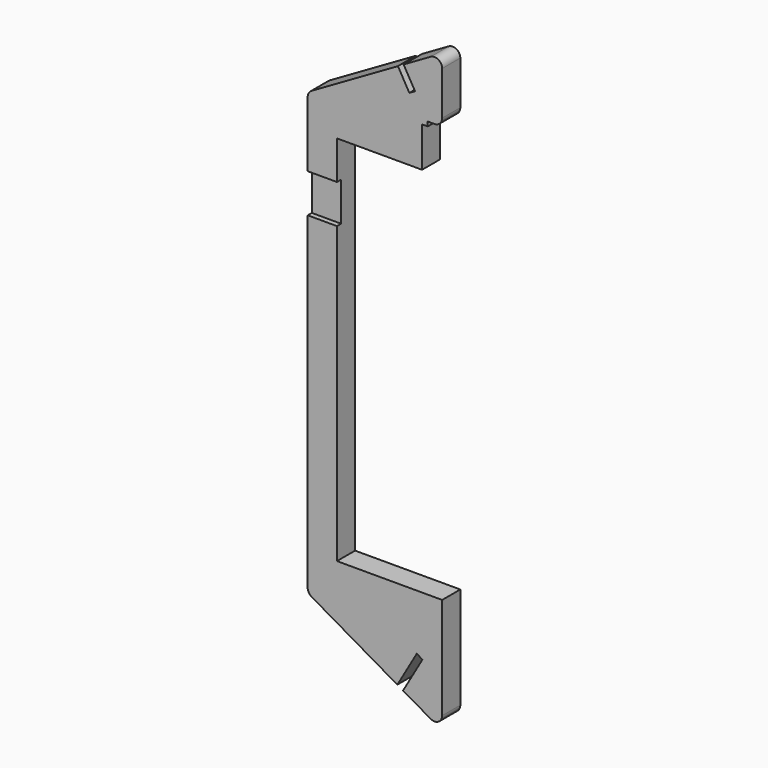
from build123d import *

# Parameters (mm, degrees)
F1_DEPTH  = 16.1798
F2_W      = 14.6956490017
F2_H      = 39.0100460752
F3_DEPTH  = 25.4
F4_W      = 7.289106492
F4_H      = 24.3518359493
F5_DEPTH  = 6.0198
F6_W      = 0.4318
F6_H      = 1.4841509983
F7_DEPTH  = 2.54
F8_W      = 1.707770396
F8_H      = 26.8365105148
F9_DEPTH  = 5.8674
F10_W     = 4.3080397882
F10_H     = 25.773898873
F11_DEPTH = 8.382
F12_W     = 0.4299804568
F12_H     = 1.4841509983
F13_DEPTH = 1.4986
F14_W     = 0.3396534594
F14_H     = 2.54
F14_W_2   = 0.0413465406
F15_DEPTH = 25.4
F16_R     = 0.5


with BuildPart() as f1:
    # F0 (on Front) → F1 (new body)
    with BuildSketch(Plane.XZ):
        Polygon((7.4940245816, -8.5250653475), (7.4940245816, 30.4849807278), (-1.3047935208, 25.4049807278), (-1.3047935208, -3.4450653475), align=None)
    extrude(amount=F1_DEPTH)

    # F2 (on face) → F3 (cut)
    with BuildSketch(Plane.YZ.offset(7.4940245816)):
        with Locations((-8.8319754991, 10.9799576901)):
            Rectangle(F2_W, F2_H)
    extrude(amount=-F3_DEPTH, mode=Mode.SUBTRACT)

    # F4 (on face) → F5 (cut)
    with BuildSketch(Plane.XZ):
        with Locations((4.2547506746, 11.1802831525)):
            Rectangle(F4_W, F4_H)
    extrude(amount=F5_DEPTH, mode=Mode.SUBTRACT)

    # F6 (on face) → F7 (cut)
    with BuildSketch(Plane(origin=(-1.8179554345, 0, -3.1487911785), x_dir=(0.8660254038, 0, -0.5), z_dir=(-0.5, 0, -0.8660254038))):
        with Locations((7.5819472408, 0.7420754991)):
            Rectangle(F6_W, F6_H)
    extrude(amount=-F7_DEPTH, mode=Mode.SUBTRACT)

    # F8 (on Front) → F9 (cut)
    with BuildSketch(Plane.XZ):
        with Locations((7.0332919713, 12.55759981)):
            Rectangle(F8_W, F8_H)
    extrude(amount=F9_DEPTH, mode=Mode.SUBTRACT)

    # F10 (on Front) → F11 (cut)
    with BuildSketch(Plane.XZ):
        with Locations((8.7046686094, 13.3732402755)):
            Rectangle(F10_W, F10_H)
    extrude(amount=F11_DEPTH, mode=Mode.SUBTRACT)

    # F12 (on face) → F13 (cut)
    with BuildSketch(Plane(origin=(-11.3268777267, 0, 19.6187277137), x_dir=(0.8660254038, 0, 0.5), z_dir=(-0.5, 0, 0.8660254038))):
        with Locations((18.6048597097, -0.7420754991)):
            Rectangle(F12_W, F12_H)
    extrude(amount=-F13_DEPTH, mode=Mode.SUBTRACT)

    # F14 (on face) → F15 (cut)
    with BuildSketch(Plane.YZ.offset(0.6101974286)):
        with Locations((-1.3143242686, 19.5710362089)):
            Rectangle(F14_W, F14_H)
        with Locations((-1.5048242686, 19.5710362089)):
            Rectangle(F14_W_2, F14_H)
    extrude(amount=-F15_DEPTH, mode=Mode.SUBTRACT)

    # F16
    f16_edges = [f1.edges().sort_by_distance(p)[0] for p in [
        (7.494025, -0.742075, 30.484981),
        (7.494025, -0.742075, -8.525065),
        (-1.304794, -0.742075, -3.445065),
        (-1.304794, -0.742075, 25.404981),
        (7.494025, -0.742075, 26.26019),
    ]]
    fillet(f16_edges, radius=F16_R)


solid = f1.part
